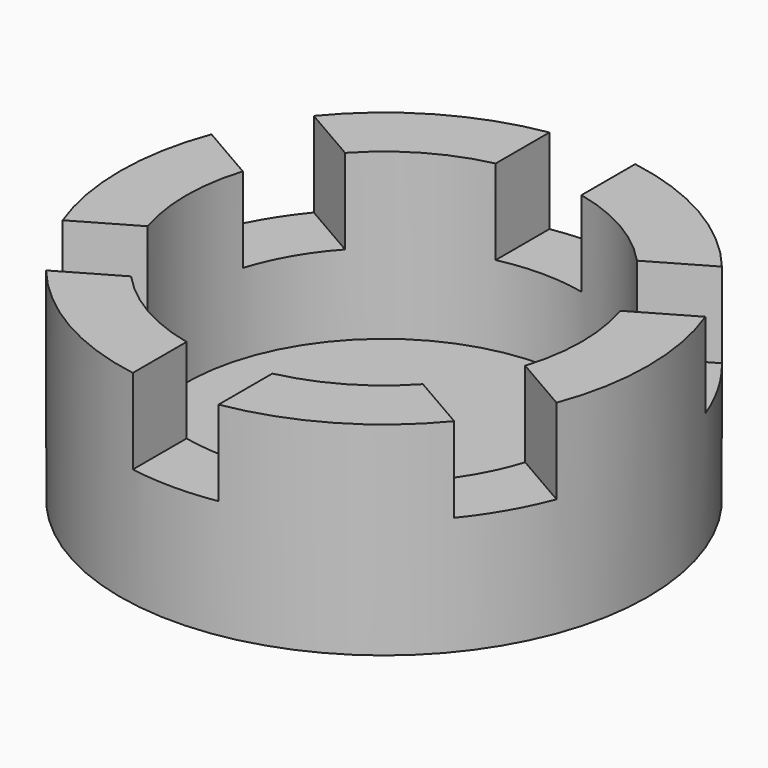
from build123d import *

# Parameters (mm, degrees)
F0_R            = 40
F0_R_2          = 30
F1_DEPTH        = 25
F3_DEPTH        = 12.8905829042
F3_COPIES_COUNT = 6
F5_R            = 40
F5_R_2          = 30
F6_DEPTH        = 5.8128256351


# Not quite as in the source:
# - a pattern or mirror of a feature is missing from the dataset's text; its kind, count and spacing are read off the source's solid


with BuildPart() as f1:
    # F0 (on Top) → F1 (new body)
    with BuildSketch(Plane.XY):
        Circle(F0_R)
        Circle(F0_R_2, mode=Mode.SUBTRACT)
    extrude(amount=F1_DEPTH)

    # F2 (on face) → F3 (cut)
    with BuildSketch(Plane.XY.offset(25)):
        with BuildLine():
            Line((6.5, 29.2873692912), (6.5, 39.4683417437))
            ThreePointArc((6.5, 39.4683417437), (3.2608534351, 39.8668638706), (0, 40))
            ThreePointArc((0, 40), (-3.2608534351, 39.8668638706), (-6.5, 39.4683417437))
            Line((-6.5, 39.4683417437), (-6.5, 29.2873692912))
            ThreePointArc((-6.5, 29.2873692912), (-3.2694740604, 29.8213101551), (0, 30))
            ThreePointArc((0, 30), (3.2694740604, 29.8213101551), (6.5, 29.2873692912))
        make_face()
    f3 = extrude(amount=-F3_DEPTH, mode=Mode.SUBTRACT)

    # F3_copies: F3 ×6 about axis
    f3_copies_axis = Axis((0, 0, 0), (0, 0, 1))
    for i in range(1, F3_COPIES_COUNT):
        add(f3.rotate(f3_copies_axis, i * 360 / F3_COPIES_COUNT), mode=Mode.SUBTRACT)

    # F5 (on face) → F6 (join)
    with BuildSketch(Plane(origin=(0, 0, 0), x_dir=(1, 0, 0), z_dir=(0, 0, -1))):
        Circle(F5_R)
        Circle(F5_R_2, mode=Mode.SUBTRACT)
        Circle(F5_R)
    extrude(amount=F6_DEPTH)


solid = f1.part
